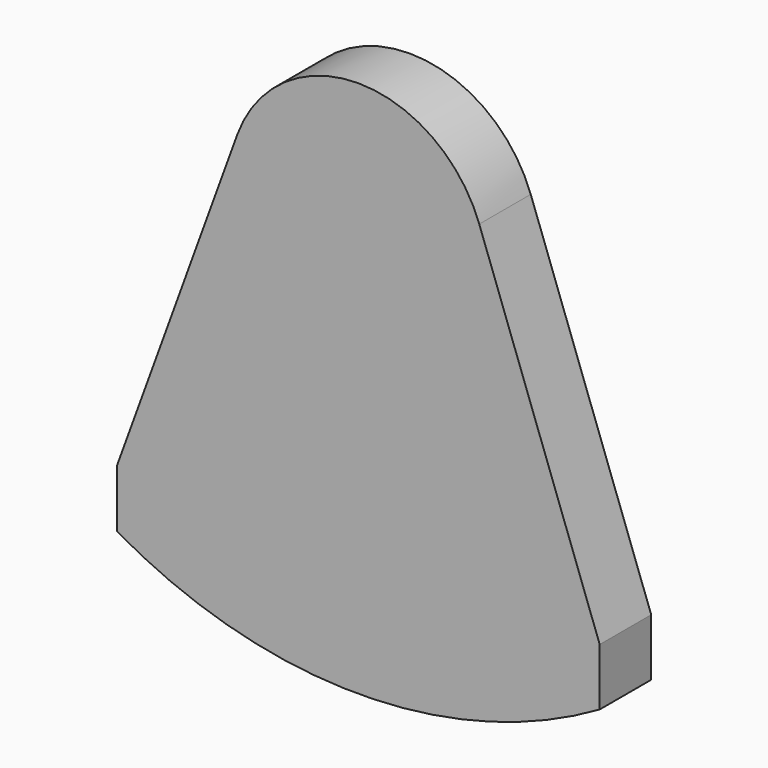
from build123d import *

# Parameters (mm, degrees)
F2_DEPTH = 20


with BuildPart() as f2:
    # F1 (on Front) → F2 (new body)
    with BuildSketch(Plane.XZ):
        with BuildLine():
            ThreePointArc((37.5877048314, 128.680805733), (0, 155), (-37.5877048314, 128.680805733))
            Line((-37.5877048314, 128.680805733), (-75, 25.8913695474))
            Line((-75, 25.8913695474), (-75, 8.0961894323))
            ThreePointArc((-75, 8.0961894323), (0, -12), (75, 8.0961894323))
            Line((75, 8.0961894323), (75, 25.8913695474))
            Line((75, 25.8913695474), (37.5877048314, 128.680805733))
        make_face()
    extrude(amount=-F2_DEPTH)


solid = f2.part
